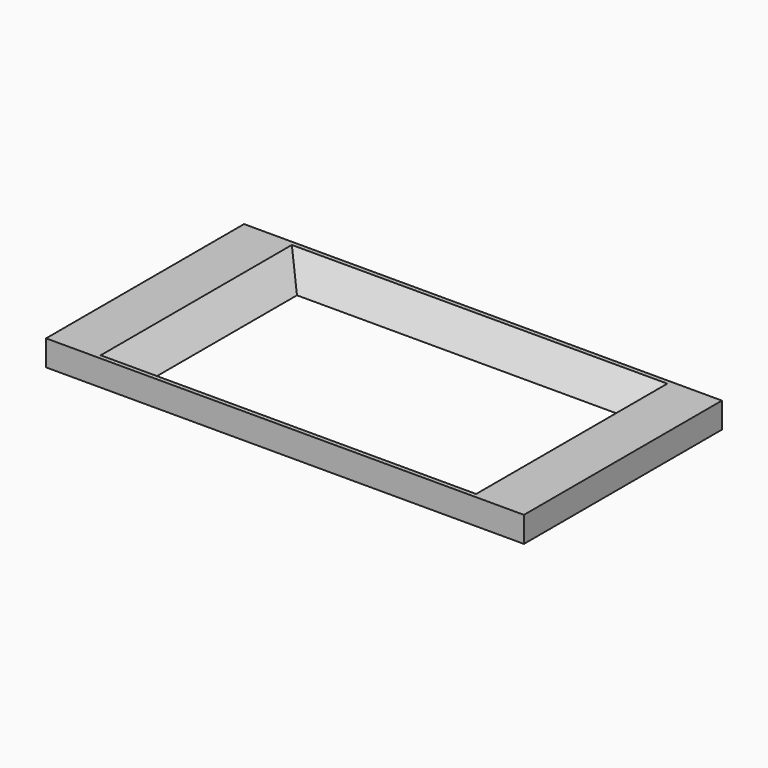
from build123d import *

# Parameters (mm, degrees)
F0_W     = 355.6
F0_H     = 184.15
F0_W_2   = 241.3
F0_H_2   = 139.7
F1_DEPTH = 19.05
F2_SIZE  = 19.04999


# Not quite as in the source:
# - a fillet or chamfer is up to 0.001 mm smaller than in the source, because OpenCascade refuses the exact size


with BuildPart() as f1:
    # F0 (on Top) → F1 (new body)
    with BuildSketch(Plane.XY):
        Rectangle(F0_W, F0_H)
        Rectangle(F0_W_2, F0_H_2, mode=Mode.SUBTRACT)
    extrude(amount=F1_DEPTH)

    # F2 (size 19.05 in the source; OpenCascade refuses exactly that, so slightly less here)
    f2_edges = [f1.edges().sort_by_distance(p)[0] for p in [
        (-120.65, 0, 19.05),
        (0, 69.85, 19.05),
        (120.65, 0, 19.05),
        (0, -69.85, 19.05),
    ]]
    chamfer(f2_edges, length=F2_SIZE)


solid = f1.part
